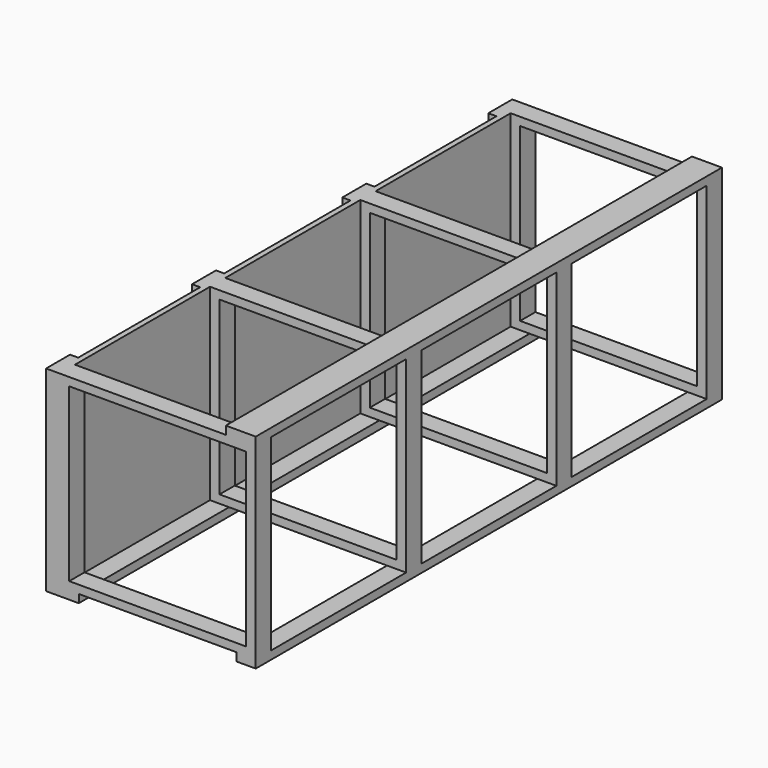
from build123d import *

# Parameters (mm, degrees)
F1_DEPTH  = 2717.8
F2_W      = 914.4
F2_H      = 787.4
F3_DEPTH  = 38.1
F4_W      = 44.45
F4_H      = 88.9
F5_DEPTH  = 800.1
F6_W      = 88.9
F6_H      = 38.1
F7_DEPTH  = 914.4
F8_W      = 139.7
F8_H      = 38.1
F9_DEPTH  = 2717.8
F10_W     = 139.7
F10_H     = 914.4
F11_DEPTH = 63.5
F12_W     = 25.4
F12_H     = 2717.8
F13_DEPTH = 914.4


with BuildPart() as f1:
    # F0 (on Front) → F1 (new body)
    with BuildSketch(Plane.XZ):
        Polygon((0, 76.2), (0, 0), (88.9, 0), (88.9, 38.1), (825.5, 38.1), (825.5, 0), (914.4, 0), (914.4, 76.2), align=None)
    extrude(amount=F1_DEPTH)

    # F2 (on face) → F3 (cut)
    with BuildSketch(Plane.XY.offset(76.2)):
        with Locations((457.2, -2235.2)):
            Rectangle(F2_W, F2_H)
        with Locations((457.2, -1358.9)):
            Rectangle(F2_W, F2_H)
        with Locations((457.2, -482.6)):
            Rectangle(F2_W, F2_H)
    extrude(amount=-F3_DEPTH, mode=Mode.SUBTRACT)

    # F4 (on face) → F5 (join)
    with BuildSketch(Plane.XY.offset(76.2)):
        with Locations((892.175, -44.45)):
            Rectangle(F4_W, F4_H)
        with Locations((22.225, -44.45)):
            Rectangle(F4_W, F4_H)
        with Locations((22.225, -920.75)):
            Rectangle(F4_W, F4_H)
        with Locations((892.175, -920.75)):
            Rectangle(F4_W, F4_H)
        with Locations((892.175, -1797.05)):
            Rectangle(F4_W, F4_H)
        with Locations((22.225, -1797.05)):
            Rectangle(F4_W, F4_H)
        with Locations((22.225, -2673.35)):
            Rectangle(F4_W, F4_H)
        with Locations((892.175, -2673.35)):
            Rectangle(F4_W, F4_H)
    extrude(amount=F5_DEPTH)

    # F6 (on face) → F7 (join)
    with BuildSketch(Plane.YZ.offset(914.4)):
        with Locations((-2673.35, 895.35)):
            Rectangle(F6_W, F6_H)
        with Locations((-44.45, 895.35)):
            Rectangle(F6_W, F6_H)
        with Locations((-1797.05, 895.35)):
            Rectangle(F6_W, F6_H)
        with Locations((-920.75, 895.35)):
            Rectangle(F6_W, F6_H)
    extrude(amount=-F7_DEPTH)

    # F8 (on face) → F9 (join)
    with BuildSketch(Plane.XZ.offset(2717.8)):
        with Locations((844.55, 933.45)):
            Rectangle(F8_W, F8_H)
    extrude(amount=-F9_DEPTH)

    # F10 (on face) → F11 (join)
    with BuildSketch(Plane(origin=(0, 0, 0), x_dir=(0, -1, 0), z_dir=(-1, 0, 0))):
        with Locations((69.85, 457.2)):
            Rectangle(F10_W, F10_H)
        with Locations((2647.95, 457.2)):
            Rectangle(F10_W, F10_H)
        with Locations((920.75, 457.2)):
            Rectangle(F10_W, F10_H)
        with Locations((1797.05, 457.2)):
            Rectangle(F10_W, F10_H)
    extrude(amount=F11_DEPTH)

    # F12 (on face) → F13 (join)
    with BuildSketch(Plane.XY.offset(914.4)):
        with Locations((-12.7, -1358.9)):
            Rectangle(F12_W, F12_H)
    extrude(amount=-F13_DEPTH)


solid = f1.part
